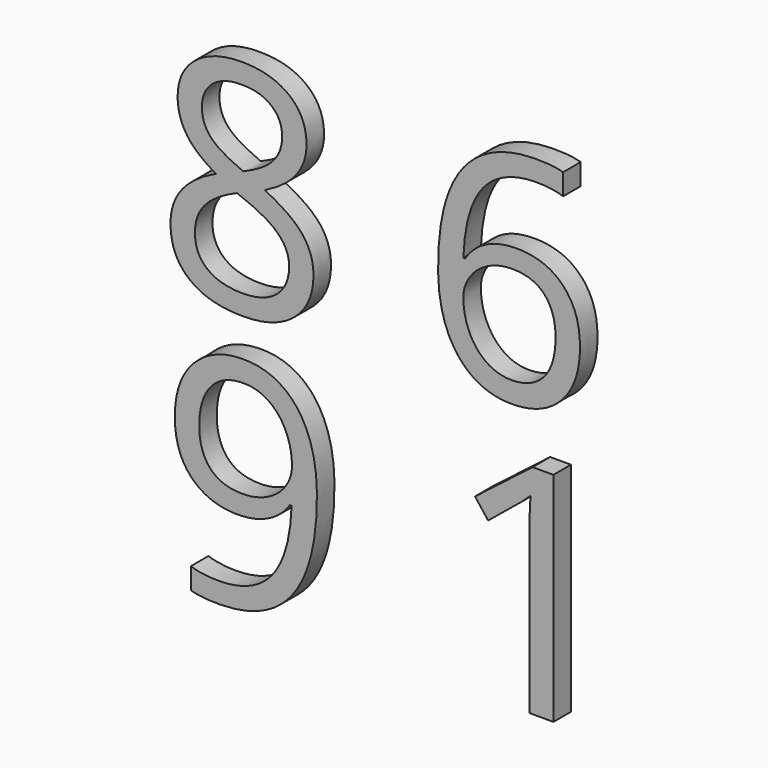
from build123d import *

# Parameters (mm, degrees)
F0_TEXT_SIZE = 88.1944444444
F1_DEPTH     = 6.35


# Not quite as in the source:
# - Text() gives the source's letters only with a copy of the font that has no kerning and outlines rounded to 1/6400 em; it was checked with that copy


with BuildPart() as f1:
    # F0 (on Front) → F1 (new body)
    with BuildSketch(Plane.XZ):
        with Locations((-64.475288389, 4.4505477422)):
            Text('8', F0_TEXT_SIZE, font='Open Sans', text_align=(TextAlign.LEFT, TextAlign.BOTTOM))
        with Locations((12.3963251325, 7.4064416622)):
            Text('6', F0_TEXT_SIZE, font='Open Sans', text_align=(TextAlign.LEFT, TextAlign.BOTTOM))
        with Locations((-63.3076519337, -71.1588258751)):
            Text('9', F0_TEXT_SIZE, font='Open Sans', text_align=(TextAlign.LEFT, TextAlign.BOTTOM))
        with Locations((20.0379335808, -70.5515523405)):
            Text('1', F0_TEXT_SIZE, font='Open Sans', text_align=(TextAlign.LEFT, TextAlign.BOTTOM))
    extrude(amount=F1_DEPTH)


solid = f1.part
